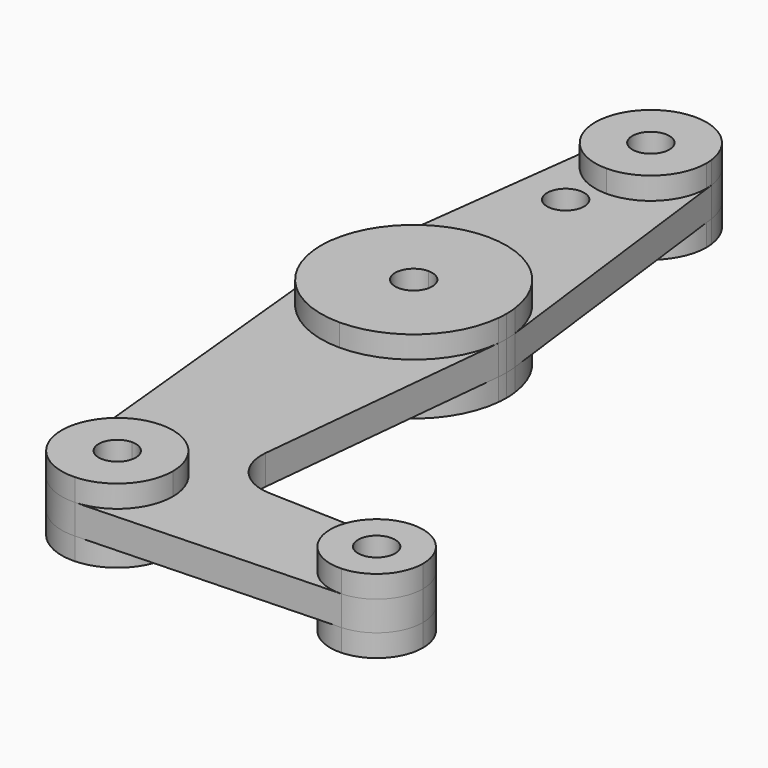
from build123d import *

# Parameters (mm, degrees)
F1_DEPTH = 6.35
F0_R     = 3.175
F2_DEPTH = 2.54


with BuildPart() as f1:
    # F0 (on Top) → F1 (new body, symmetric)
    with BuildSketch(Plane.XY):
        with BuildLine():
            ThreePointArc((-18.927548, 83.105366), (-16.621005, 75.614546), (-9.477255, 72.389741))
            ThreePointArc((-9.477255, 72.389741), (-2.742063, 75.179549), (0.047745, 81.914741))
            ThreePointArc((0.047745, 81.914741), (0.02905, 82.511224), (-0.026962, 83.105366))
            ThreePointArc((-0.026962, 83.105366), (-9.477255, 91.439741), (-18.927548, 83.105366))
        make_face()
        with BuildLine():
            ThreePointArc((-6.302255, 81.914741), (-7.232191, 79.669677), (-9.477255, 78.739741))
            ThreePointArc((-9.477255, 78.739741), (-11.722319, 84.159805), (-6.302255, 81.914741))
        make_face(mode=Mode.SUBTRACT)
    extrude(amount=F1_DEPTH, both=True)


with BuildPart() as f1b:
    # F0 (on Top) → F1, piece 2 (new body, symmetric)
    with BuildSketch(Plane.XY):
        with BuildLine():
            Line((-9.477255, 34.289741), (-9.477255, 46.989741))
            ThreePointArc((-9.477255, 46.989741), (-19.977581, 43.020991), (-25.227744, 33.099116))
            ThreePointArc((-25.227744, 33.099116), (-25.350999, 31.314446), (-25.272681, 29.527241))
            ThreePointArc((-25.272681, 29.527241), (-20.126529, 19.341526), (-9.477255, 15.239741))
            Line((-9.477255, 15.239741), (-9.477255, 27.939741))
            ThreePointArc((-9.477255, 27.939741), (-12.652255, 31.114741), (-9.477255, 34.289741))
        make_face()
        with BuildLine():
            ThreePointArc((6.273233, 33.099116), (1.02307, 43.020991), (-9.477255, 46.989741))
            Line((-9.477255, 46.989741), (-9.477255, 34.289741))
            ThreePointArc((-9.477255, 34.289741), (-7.232191, 33.359805), (-6.302255, 31.114741))
            ThreePointArc((-6.302255, 31.114741), (-7.232191, 28.869677), (-9.477255, 27.939741))
            Line((-9.477255, 27.939741), (-9.477255, 15.239741))
            ThreePointArc((-9.477255, 15.239741), (1.172018, 19.341526), (6.31817, 29.527241))
            ThreePointArc((6.31817, 29.527241), (6.377839, 30.319994), (6.397745, 31.114741))
            ThreePointArc((6.397745, 31.114741), (6.366586, 32.10888), (6.273233, 33.099116))
        make_face()
    extrude(amount=F1_DEPTH, both=True)


with BuildPart() as f1c:
    # F0 (on Top) → F1, piece 3 (new body, symmetric)
    with BuildSketch(Plane.XY):
        with BuildLine():
            ThreePointArc((-9.477255, -22.860259), (-16.541184, -25.995695), (-18.954511, -33.337759))
            ThreePointArc((-18.954511, -33.337759), (-15.739639, -39.562179), (-9.137077, -41.904183))
            ThreePointArc((-9.137077, -41.904183), (-2.622847, -38.999087), (0.047745, -32.385259))
            Line((0.047745, -32.385259), (-6.302255, -32.385259))
            ThreePointArc((-6.302255, -32.385259), (-11.722319, -34.630323), (-9.477255, -29.210259))
            Line((-9.477255, -29.210259), (-9.477255, -22.860259))
        make_face()
        with BuildLine():
            ThreePointArc((0.047745, -32.385259), (-2.742063, -25.650067), (-9.477255, -22.860259))
            Line((-9.477255, -22.860259), (-9.477255, -29.210259))
            ThreePointArc((-9.477255, -29.210259), (-7.232191, -30.140195), (-6.302255, -32.385259))
            Line((-6.302255, -32.385259), (0.047745, -32.385259))
        make_face()
    extrude(amount=F1_DEPTH, both=True)


with BuildPart() as f1d:
    # F0 (on Top) → F1, piece 4 (new body, symmetric)
    with BuildSketch(Plane.XY):
        with BuildLine():
            ThreePointArc((27.035245, -32.385259), (29.461222, -38.097266), (35.256227, -40.317695))
            ThreePointArc((35.256227, -40.317695), (40.684752, -37.896782), (42.910245, -32.385259))
            ThreePointArc((42.910245, -32.385259), (40.684752, -26.873736), (35.256227, -24.452823))
            ThreePointArc((35.256227, -24.452823), (29.461222, -26.673252), (27.035245, -32.385259))
        make_face()
        with BuildLine():
            ThreePointArc((38.147745, -32.385259), (34.972745, -35.560259), (31.797745, -32.385259))
            ThreePointArc((31.797745, -32.385259), (34.972745, -29.210259), (38.147745, -32.385259))
        make_face(mode=Mode.SUBTRACT)
    extrude(amount=F1_DEPTH, both=True)


with BuildPart() as f2:
    # F0 (on Top) → F2 (new body, symmetric)
    with BuildSketch(Plane.XY):
        with BuildLine():
            ThreePointArc((-18.927548, 83.105366), (-16.621005, 75.614546), (-9.477255, 72.389741))
            ThreePointArc((-9.477255, 72.389741), (-2.742063, 75.179549), (0.047745, 81.914741))
            ThreePointArc((0.047745, 81.914741), (0.02905, 82.511224), (-0.026962, 83.105366))
            ThreePointArc((-0.026962, 83.105366), (-9.477255, 91.439741), (-18.927548, 83.105366))
        make_face()
        with BuildLine():
            ThreePointArc((-6.302255, 81.914741), (-7.232191, 79.669677), (-9.477255, 78.739741))
            ThreePointArc((-9.477255, 78.739741), (-11.722319, 84.159805), (-6.302255, 81.914741))
        make_face(mode=Mode.SUBTRACT)
        with BuildLine():
            ThreePointArc((0.047745, 81.914741), (-2.742063, 75.179549), (-9.477255, 72.389741))
            Line((-9.477255, 72.389741), (-9.477255, 67.639941))
            Line((-9.477255, 67.639941), (-9.477255, 46.989741))
            ThreePointArc((-9.477255, 46.989741), (1.02307, 43.020991), (6.273233, 33.099116))
            Line((6.273233, 33.099116), (-0.026962, 83.105366))
            ThreePointArc((-0.026962, 83.105366), (0.02905, 82.511224), (0.047745, 81.914741))
        make_face()
        with BuildLine():
            Line((-9.477255, 67.639941), (-9.477255, 72.389741))
            ThreePointArc((-9.477255, 72.389741), (-16.621005, 75.614546), (-18.927548, 83.105366))
            Line((-18.927548, 83.105366), (-25.227744, 33.099116))
            ThreePointArc((-25.227744, 33.099116), (-19.977581, 43.020991), (-9.477255, 46.989741))
            Line((-9.477255, 46.989741), (-9.477255, 67.639941))
        make_face()
        with Locations((-12.652255, 67.639941)):
            Circle(F0_R, mode=Mode.SUBTRACT)
        with BuildLine():
            ThreePointArc((6.273233, 33.099116), (1.02307, 43.020991), (-9.477255, 46.989741))
            Line((-9.477255, 46.989741), (-9.477255, 34.289741))
            ThreePointArc((-9.477255, 34.289741), (-7.232191, 33.359805), (-6.302255, 31.114741))
            ThreePointArc((-6.302255, 31.114741), (-7.232191, 28.869677), (-9.477255, 27.939741))
            Line((-9.477255, 27.939741), (-9.477255, 15.239741))
            ThreePointArc((-9.477255, 15.239741), (1.172018, 19.341526), (6.31817, 29.527241))
            ThreePointArc((6.31817, 29.527241), (6.377839, 30.319994), (6.397745, 31.114741))
            ThreePointArc((6.397745, 31.114741), (6.366586, 32.10888), (6.273233, 33.099116))
        make_face()
        with BuildLine():
            Line((-9.477255, 34.289741), (-9.477255, 46.989741))
            ThreePointArc((-9.477255, 46.989741), (-19.977581, 43.020991), (-25.227744, 33.099116))
            ThreePointArc((-25.227744, 33.099116), (-25.350999, 31.314446), (-25.272681, 29.527241))
            ThreePointArc((-25.272681, 29.527241), (-20.126529, 19.341526), (-9.477255, 15.239741))
            Line((-9.477255, 15.239741), (-9.477255, 27.939741))
            ThreePointArc((-9.477255, 27.939741), (-12.652255, 31.114741), (-9.477255, 34.289741))
        make_face()
        with BuildLine():
            ThreePointArc((-9.477255, 15.239741), (-20.126529, 19.341526), (-25.272681, 29.527241))
            Line((-25.272681, 29.527241), (-18.954511, -33.337759))
            ThreePointArc((-18.954511, -33.337759), (-16.541184, -25.995695), (-9.477255, -22.860259))
            Line((-9.477255, -22.860259), (-9.477255, 15.239741))
        make_face()
        with BuildLine():
            ThreePointArc((6.31817, 29.527241), (1.172018, 19.341526), (-9.477255, 15.239741))
            Line((-9.477255, 15.239741), (-9.477255, -22.860259))
            ThreePointArc((-9.477255, -22.860259), (-2.742063, -25.650067), (0.047745, -32.385259))
            Line((0.047745, -32.385259), (27.035245, -32.385259))
            ThreePointArc((27.035245, -32.385259), (29.461222, -26.673252), (35.256227, -24.452823))
            Line((35.256227, -24.452823), (9.490345, -23.532025))
            ThreePointArc((9.490345, -23.532025), (3.783945, -20.8139), (1.863931, -14.791877))
            Line((1.863931, -14.791877), (6.31817, 29.527241))
        make_face()
        with BuildLine():
            ThreePointArc((-9.477255, -22.860259), (-16.541184, -25.995695), (-18.954511, -33.337759))
            ThreePointArc((-18.954511, -33.337759), (-15.739639, -39.562179), (-9.137077, -41.904183))
            ThreePointArc((-9.137077, -41.904183), (-2.622847, -38.999087), (0.047745, -32.385259))
            Line((0.047745, -32.385259), (-6.302255, -32.385259))
            ThreePointArc((-6.302255, -32.385259), (-11.722319, -34.630323), (-9.477255, -29.210259))
            Line((-9.477255, -29.210259), (-9.477255, -22.860259))
        make_face()
        with BuildLine():
            ThreePointArc((0.047745, -32.385259), (-2.622847, -38.999087), (-9.137077, -41.904183))
            Line((-9.137077, -41.904183), (35.256227, -40.317695))
            ThreePointArc((35.256227, -40.317695), (29.461222, -38.097266), (27.035245, -32.385259))
            Line((27.035245, -32.385259), (0.047745, -32.385259))
        make_face()
        with BuildLine():
            ThreePointArc((27.035245, -32.385259), (29.461222, -38.097266), (35.256227, -40.317695))
            ThreePointArc((35.256227, -40.317695), (40.684752, -37.896782), (42.910245, -32.385259))
            ThreePointArc((42.910245, -32.385259), (40.684752, -26.873736), (35.256227, -24.452823))
            ThreePointArc((35.256227, -24.452823), (29.461222, -26.673252), (27.035245, -32.385259))
        make_face()
        with BuildLine():
            ThreePointArc((38.147745, -32.385259), (34.972745, -35.560259), (31.797745, -32.385259))
            ThreePointArc((31.797745, -32.385259), (34.972745, -29.210259), (38.147745, -32.385259))
        make_face(mode=Mode.SUBTRACT)
    extrude(amount=F2_DEPTH, both=True)


solid = Compound([f1.part, f1b.part, f1c.part, f1d.part, f2.part])
